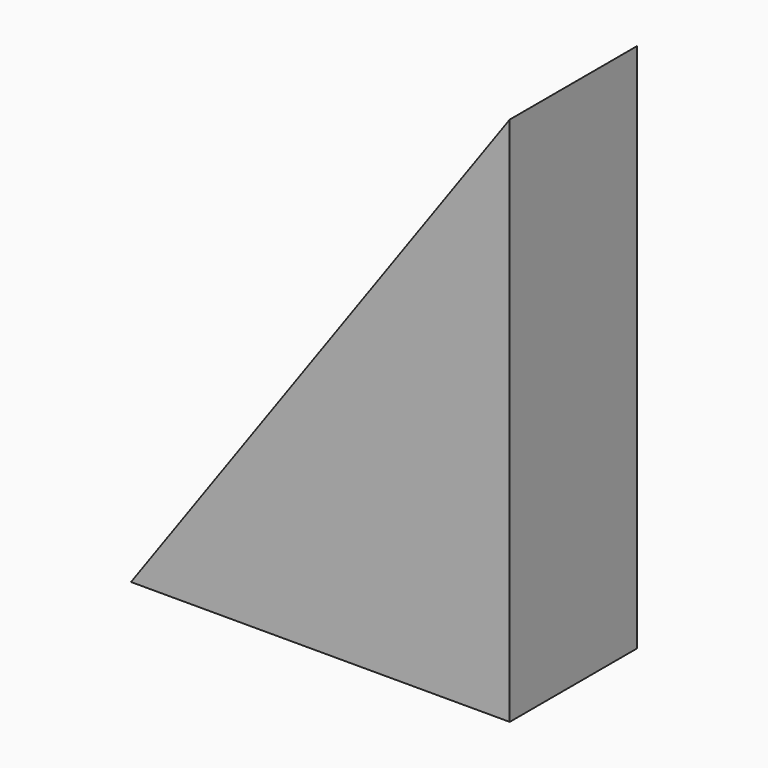
from build123d import *

# Parameters (mm, degrees)
F0_W     = 14.2837
F0_H     = 6
F1_DEPTH = 20
F2_SIZE2 = 19.99999
F2_SIZE  = 14.28369


# Not quite as in the source:
# - a fillet or chamfer is up to 0.001 mm smaller than in the source, because OpenCascade refuses the exact size


with BuildPart() as f1:
    # F0 (on Top) → F1 (new body)
    with BuildSketch(Plane.XY):
        Rectangle(F0_W, F0_H)
    extrude(amount=F1_DEPTH)

    # F2 (size 14.2837 and 20 in the source; OpenCascade refuses exactly that, so slightly less here)
    f2_edges = [f1.edges().sort_by_distance(p)[0] for p in [
        (-7.14185, 0, 20),
    ]]
    f2_side = f1.faces().sort_by_distance((0, 0, 20))[0]
    chamfer(f2_edges, length=F2_SIZE, length2=F2_SIZE2, reference=f2_side)


solid = f1.part
